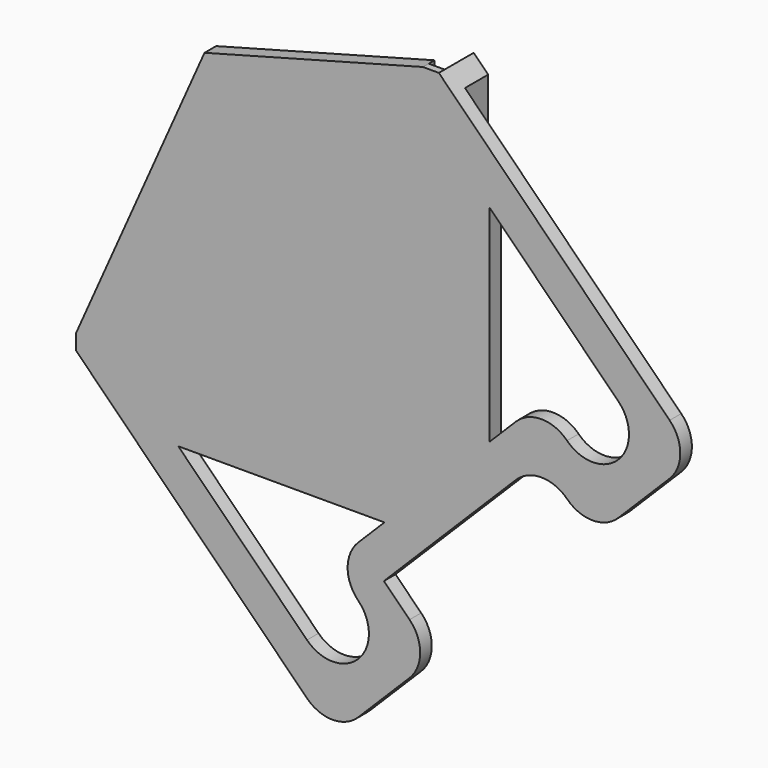
from build123d import *

# Parameters (mm, degrees)
F1_DEPTH = 2
F3_DEPTH = 4
F5_DEPTH = 25
F6_R     = 4.99999
F8_DEPTH = 1


# Not quite as in the source:
# - a fillet or chamfer is up to 0.001 mm smaller than in the source, because OpenCascade refuses the exact size


with BuildPart() as f1:
    # F0 (on Front) → F1 (new body)
    with BuildSketch(Plane.XZ):
        Polygon((-50, 2.2), (-50, 0), (-14.6446609407, -35.3553390593), (-0.5025253169, -21.2132034356), (-7.5735931288, -14.1421356237), (14.1421356237, 7.5735931288), (21.2132034356, 0.5025253169), (35.3553390593, 14.6446609407), (0, 50), (-2.2, 50), (-2.2, 2.2), align=None)
        Polygon((-32.3101722444, 41.9320036632), (-50, 2.2), (-2.2, 2.2), (-2.2, 50), align=None)
    extrude(amount=F1_DEPTH)

    # F2 (on face) → F3 (join)
    with BuildSketch(Plane(origin=(0, 0, 0), x_dir=(-1, 0, 0), z_dir=(0, 1, 0))):
        Polygon((0, 0), (0, 50), (-2, 48), (-2, -2), (48, -2), (50, 0), align=None)
        Polygon((4.2, 45.3229968935), (2.2, 45.8588952784), (2.2, 2.2), (45.621454886, 2.2), (44.7309975154, 4.2), (4.2, 4.2), align=None)
    extrude(amount=F3_DEPTH)

    # F4 (on face) → F5 (cut)
    with BuildSketch(Plane(origin=(0, 0, 0), x_dir=(-1, 0, 0), z_dir=(0, 1, 0))):
        Polygon((7.5735934344, -21.2132034356), (14.6446609407, -28.2842709419), (35.9289316665, -7.0000002161), (7.5025258386, -7.0000002161), (14.6446612462, -14.1421356237), align=None)
        Polygon((-14.1421356237, 14.6446612462), (-7.0000002161, 7.5025258386), (-7.0000002161, 35.9289316665), (-28.2842709419, 14.6446609407), (-21.2132034356, 7.5735934344), align=None)
    extrude(amount=-F5_DEPTH, mode=Mode.SUBTRACT)

    # F6 (radius 5 in the source; OpenCascade refuses exactly that, so slightly less here)
    f6_edges = [f1.edges().sort_by_distance(p)[0] for p in [
        (35.355339, -1, 14.644661),
        (21.213203, -1, 0.502525),
        (-14.644661, -1, -35.355339),
        (-0.502525, -1, -21.213203),
        (-14.644661, -1, -14.142136),
        (14.142136, -1, 14.644661),
        (14.142136, -1, 7.573593),
        (21.213203, -1, 7.573593),
        (28.284271, -1, 14.644661),
        (-14.644661, -1, -28.284271),
        (-7.573593, -1, -21.213203),
    ]]
    fillet(f6_edges, radius=F6_R)

    # F7 (on face) → F8 (cut)
    with BuildSketch(Plane(origin=(0, 0, 0), x_dir=(-1, 0, 0), z_dir=(0, 1, 0))):
        Polygon((2.2, 50), (0, 50), (0, 0), (50, 0), (50, 2.2), (45.621454886, 2.2), (2.2, 2.2), (2.2, 45.8588952784), align=None)
    extrude(amount=-F8_DEPTH, mode=Mode.SUBTRACT)


solid = f1.part
